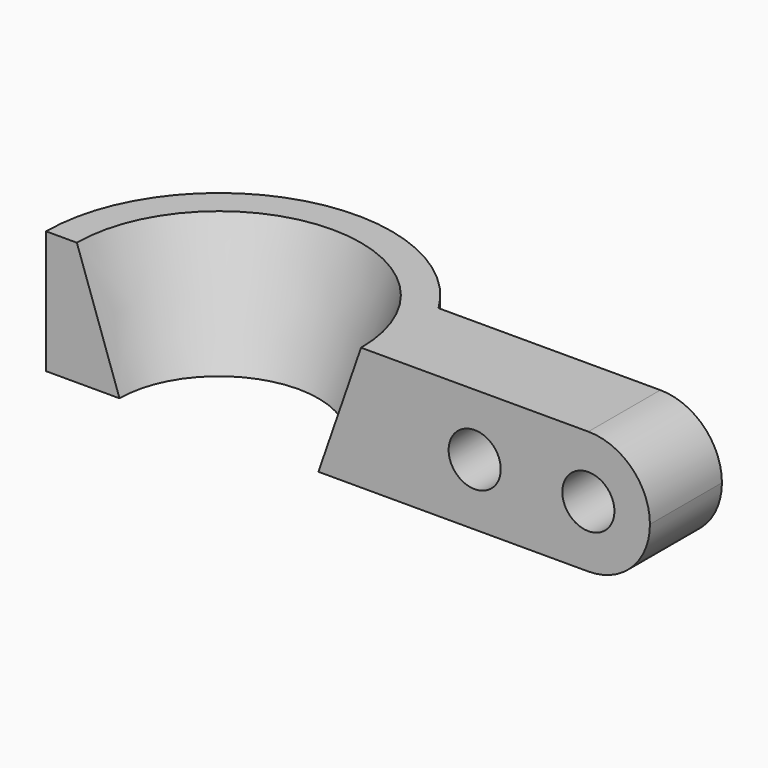
from build123d import *

# Parameters (mm, degrees)
F1_DEPTH = 52
F4_R     = 25.99999
F5_R     = 11
F6_DEPTH = 100


# Not quite as in the source:
# - a fillet or chamfer is up to 0.001 mm smaller than in the source, because OpenCascade refuses the exact size


with BuildPart() as f1:
    # F0 (on Top) → F1 (new body)
    with BuildSketch(Plane.XY):
        with BuildLine():
            ThreePointArc((62.329768169, 38), (-19.7348286497, 70.2818364741), (-73, 0))
            Line((-73, 0), (182, 0))
            Line((182, 0), (182, 38))
            Line((182, 38), (62.329768169, 38))
        make_face()
    extrude(amount=F1_DEPTH)

    # F2 (on face) → F3 (revolve, cut)
    with BuildSketch(Plane.XZ):
        Polygon((60, 52), (0, 52), (0, 0), (42, 0), align=None)
    revolve(axis=Axis((0, 0, 26), (0, 0, -1)), mode=Mode.SUBTRACT)

    # F4 (radius 26 in the source; OpenCascade refuses exactly that, so slightly less here)
    f4_edges = [f1.edges().sort_by_distance(p)[0] for p in [
        (182, 19, 52),
        (182, 19, 0),
    ]]
    fillet(f4_edges, radius=F4_R)

    # F5 (on face) → F6 (cut)
    with BuildSketch(Plane.XZ):
        with Locations((108, 26)):
            Circle(F5_R)
        with Locations((156, 26)):
            Circle(F5_R)
    extrude(amount=-F6_DEPTH, mode=Mode.SUBTRACT)


solid = f1.part
